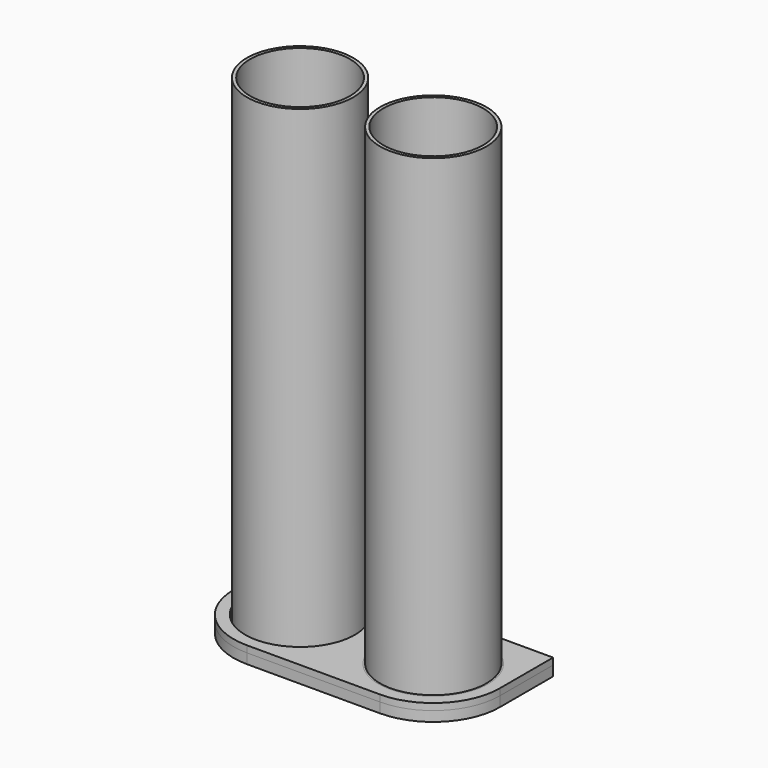
from build123d import *

# Parameters (mm, degrees)
F0_R     = 57.15
F1_DEPTH = 6.35
F2_DEPTH = 25.4
F4_DEPTH = 9.525
F5_R     = 50.8
F5_R_2   = 47.625
F6_DEPTH = 457.2
F7_DEPTH = 3.175
F8_DEPTH = 3.175
F9_DEPTH = 6.35
F10_D    = 104.775


# Not quite as in the source:
# - a feature names something its author has since deleted; it is built from what else it names


with BuildPart() as f1:
    # F0 (on Top) → F1 (new body)
    with BuildSketch(Plane.XY):
        Circle(F0_R)
    extrude(amount=F1_DEPTH)

    # F2 (cut): a face of the model
    f2_faces = [f1.faces().sort_by_distance(p)[0] for p in [
        (0, 0, 6.35),
    ]]
    extrude(f2_faces, amount=F2_DEPTH, mode=Mode.SUBTRACT)

    # F5 (on Top) → F7 (cut)
    with BuildSketch(Plane.XY):
        Circle(F5_R)
        Circle(F5_R_2, mode=Mode.SUBTRACT)
        with Locations((-127, 0)):
            Circle(F5_R)
        with Locations((-127, 0)):
            Circle(F5_R_2, mode=Mode.SUBTRACT)
    extrude(amount=F7_DEPTH, mode=Mode.SUBTRACT)


with BuildPart() as f4:
    # F3 (on Top) → F4 (new body)
    with BuildSketch(Plane.XY):
        with BuildLine():
            Line((-190.5, 63.5), (-190.5, 0))
            ThreePointArc((-190.5, 0), (-171.9012806053, -44.9012806053), (-127, -63.5))
            Line((-127, -63.5), (0, -63.5))
            ThreePointArc((0, -63.5), (44.9012806053, -44.9012806053), (63.5, 0))
            Line((63.5, 0), (63.5, 63.5))
            Line((63.5, 63.5), (-190.5, 63.5))
        make_face()
    extrude(amount=-F4_DEPTH)

    # F5 (on Top) → F8 (cut)
    with BuildSketch(Plane.XY):
        Circle(F5_R)
        Circle(F5_R_2, mode=Mode.SUBTRACT)
        with Locations((-127, 0)):
            Circle(F5_R)
        with Locations((-127, 0)):
            Circle(F5_R_2, mode=Mode.SUBTRACT)
    extrude(amount=-F8_DEPTH, mode=Mode.SUBTRACT)


with BuildPart() as f6:
    # F5 (on Top) → F6 (new body)
    with BuildSketch(Plane.XY):
        Circle(F5_R)
        Circle(F5_R_2, mode=Mode.SUBTRACT)
    extrude(amount=F6_DEPTH)


with BuildPart() as f6b:
    # F5 (on Top) → F6, piece 2 (new body)
    with BuildSketch(Plane.XY):
        with Locations((-127, 0)):
            Circle(F5_R)
        with Locations((-127, 0)):
            Circle(F5_R_2, mode=Mode.SUBTRACT)
    extrude(amount=F6_DEPTH)


with BuildPart() as f9:
    # F3 (on Top) → F9 (new body)
    with BuildSketch(Plane.XY):
        with BuildLine():
            Line((-190.5, 63.5), (-190.5, 0))
            ThreePointArc((-190.5, 0), (-171.9012806053, -44.9012806053), (-127, -63.5))
            Line((-127, -63.5), (0, -63.5))
            ThreePointArc((0, -63.5), (44.9012806053, -44.9012806053), (63.5, 0))
            Line((63.5, 0), (63.5, 63.5))
            Line((63.5, 63.5), (-190.5, 63.5))
        make_face()
    extrude(amount=F9_DEPTH)

    # F10 (through all)
    with Locations(Plane(origin=(0, 0, 0), x_dir=(1, 0, 0), z_dir=(0, 0, -1))):
        with Locations((-127, 0), (0, 0)):
            Hole(F10_D / 2)


solid = Compound([f1.part, f4.part, f6.part, f6b.part, f9.part])
